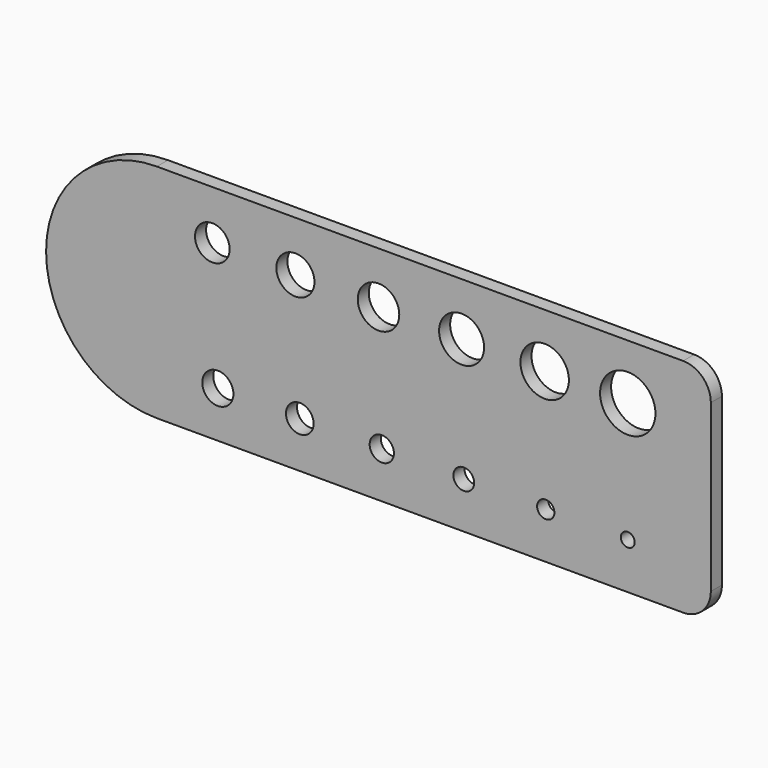
from build123d import *

# Parameters (mm, degrees)
F0_R     = 3.571875
F0_R_2   = 3.175
F0_R_3   = 2.778125
F0_R_4   = 2.38125
F0_R_5   = 1.984375
F0_R_6   = 1.5875
F0_R_7   = 3.96875
F0_R_8   = 4.365625
F0_R_9   = 4.7625
F0_R_10  = 5.159375
F0_R_11  = 5.55625
F0_R_12  = 6.35
F1_DEPTH = 3.175


# Not quite as in the source:
# - a length typed as a fraction of an inch, garbled in the dataset ("3 / 203.2 mm" for 3/8 in), is restored


with BuildPart() as f1:
    # F0 (on Front) → F1 (new body)
    with BuildSketch(Plane.XZ):
        with BuildLine():
            Line((0, 50.8), (0, 0))
            Line((0, 0), (120.65, 0))
            ThreePointArc((120.65, 0), (125.1401280605, 1.8598719395), (127, 6.35))
            Line((127, 6.35), (127, 44.45))
            ThreePointArc((127, 44.45), (125.1401280605, 48.9401280605), (120.65, 50.8))
            Line((120.65, 50.8), (0, 50.8))
        make_face()
        with Locations((13.97, 10.5871595442)):
            Circle(F0_R, mode=Mode.SUBTRACT)
        with Locations((32.766, 10.5871595442)):
            Circle(F0_R_2, mode=Mode.SUBTRACT)
        with Locations((51.562, 10.5871595442)):
            Circle(F0_R_3, mode=Mode.SUBTRACT)
        with Locations((70.358, 10.5871595442)):
            Circle(F0_R_4, mode=Mode.SUBTRACT)
        with Locations((89.154, 10.5871595442)):
            Circle(F0_R_5, mode=Mode.SUBTRACT)
        with Locations((107.95, 10.5871595442)):
            Circle(F0_R_6, mode=Mode.SUBTRACT)
        with Locations((12.7109313135, 39.5430161922)):
            Circle(F0_R_7, mode=Mode.SUBTRACT)
        with Locations((31.7587450508, 39.2544129538)):
            Circle(F0_R_8, mode=Mode.SUBTRACT)
        with Locations((50.8065587881, 38.9658097153)):
            Circle(F0_R_9, mode=Mode.SUBTRACT)
        with Locations((69.8543725254, 38.6772064769)):
            Circle(F0_R_10, mode=Mode.SUBTRACT)
        with Locations((88.9021862627, 38.3886032384)):
            Circle(F0_R_11, mode=Mode.SUBTRACT)
        with Locations((107.95, 38.1)):
            Circle(F0_R_12, mode=Mode.SUBTRACT)
        with BuildLine():
            ThreePointArc((0, 50.8), (-25.4, 25.4), (0, 0))
            Line((0, 0), (0, 50.8))
        make_face()
    extrude(amount=F1_DEPTH)


solid = f1.part
